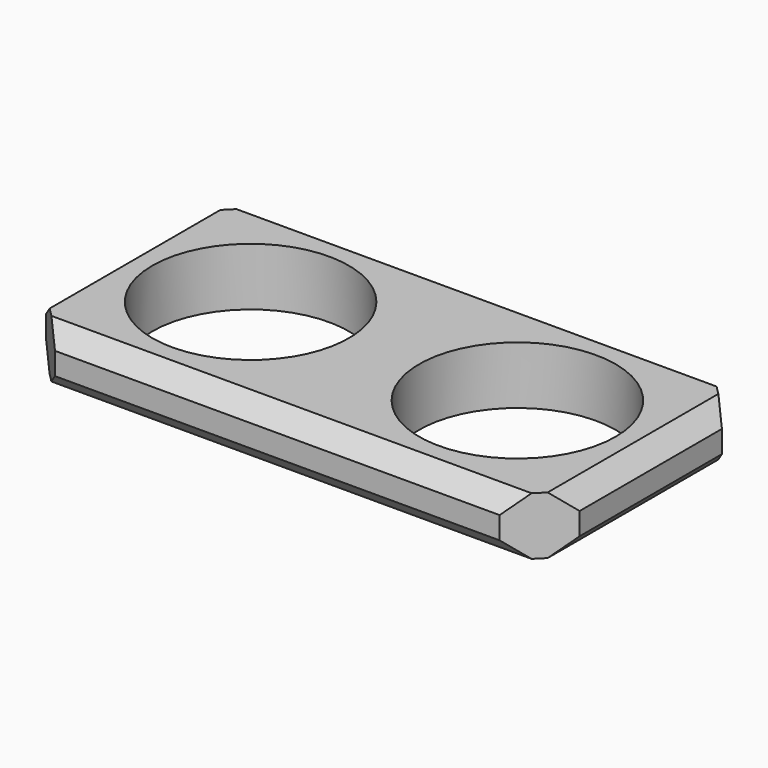
from build123d import *

# Parameters (mm, degrees)
F0_R        = 11.05
F1_DEPTH    = 6.5
F2_SIZE     = 2
F3_T1_DEPTH = 28.2168298797


# Not quite as in the source:
# - a fillet or chamfer that OpenCascade refuses, or shapes differently, is made with other operations: its cross-section is extruded or revolved along the edge and cut away or added


with BuildPart() as f1:
    # F0 (on Top) → F1 (new body)
    with BuildSketch(Plane.XY):
        Polygon((30, 0), (30, 15), (-30, 15), (-30, 0), (-30, -15), (30, -15), align=None)
        with BuildLine():
            ThreePointArc((-3.95, 0), (-15, -11.05), (-26.05, 0))
            ThreePointArc((-26.05, 0), (-15, 11.05), (-3.95, 0))
        make_face(mode=Mode.SUBTRACT)
        with Locations((15, 0)):
            Circle(F0_R, mode=Mode.SUBTRACT)
    extrude(amount=F1_DEPTH)

    # F2
    f2_edges = [f1.edges().sort_by_distance(p)[0] for p in [
        (-30, 0, 6.5),
        (-30, 0, 0),
        (0, -15, 0),
        (0, -15, 6.5),
        (0, 15, 0),
        (0, 15, 6.5),
        (30, 0, 0),
        (30, 0, 6.5),
    ]]
    chamfer(f2_edges, length=F2_SIZE)

    # F3: chamfer of 5 on 4 edges, made by hand

    # F3_s2 → F3_t1 (cut)
    with BuildSketch(Plane.XY.offset(-10.8584149398)):
        Polygon((30, 10), (25, 15), (30, 15), align=None)
        Polygon((30, -10), (25, -15), (30, -15), align=None)
        Polygon((-25, 15), (-30, 10), (-30, 15), align=None)
        Polygon((-25, -15), (-30, -10), (-30, -15), align=None)
    extrude(amount=F3_T1_DEPTH, mode=Mode.SUBTRACT)


solid = f1.part
